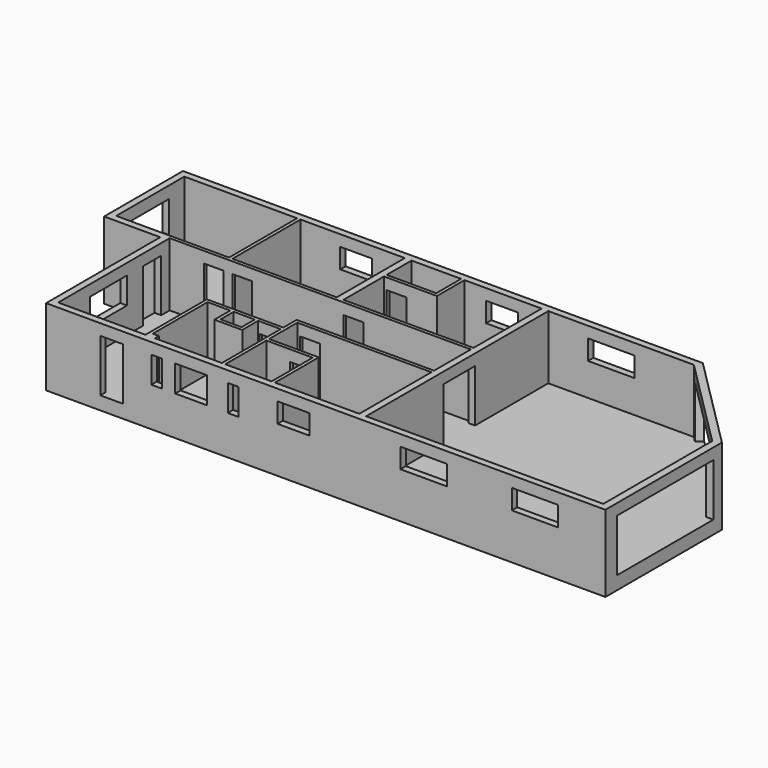
from build123d import *

# Parameters (mm, degrees)
F0_W          = 1750
F0_H          = 1938.4325688744
F0_W_2        = 796
F0_H_2        = 623
F0_W_3        = 4260
F0_H_3        = 3212
F0_W_4        = 3940
F0_W_5        = 1873
F0_H_4        = 1173
F1_DEPTH      = 2400
F1_DEPTH_BACK = 500
F2_W          = 750
F2_H          = 1980
F3_DEPTH      = 250
F4_W          = 750
F4_H          = 1980
F5_DEPTH      = 500
F6_W          = 750
F6_H          = 1980
F7_DEPTH      = 500
F8_W          = 1500
F8_H          = 1980
F9_DEPTH      = 500
F12_DEPTH     = 500
F13_W         = 750
F13_H         = 1980
F14_DEPTH     = 500
F15_W         = 1750
F15_H         = 1000
F15_W_2       = 850
F15_H_2       = 1980
F16_DEPTH     = 2374.001
F17_W         = 1750
F17_H         = 1200
F18_DEPTH     = 254.001
F19_W         = 850
F19_H         = 1980
F20_DEPTH     = 254.001
F21_W         = 400
F21_H         = 1000
F21_W_2       = 1200
F21_H_2       = 750
F21_W_3       = 1750
F22_DEPTH     = 254.001
F23_W         = 1200
F23_H         = 750
F23_W_2       = 1750
F24_DEPTH     = 254.001
F25_W         = 4294.8904704813
F25_H         = 1980
F26_DEPTH     = 2827.5745303553
F27_W         = 4540.7897551572
F27_H         = 1980
F28_DEPTH     = 283.5835903928
F29_W         = 750
F29_H         = 1980
F30_DEPTH     = 500


# Not quite as in the source:
# - a feature names something its author has since deleted; it is built from what else it names


with BuildPart() as f1:
    # F0 (on Top) → F1 (new body, two sides)
    with BuildSketch(Plane.XY) as f1_sk:
        Polygon((105.2102448428, 99.540888462), (-19524.7897551572, 99.540888462), (-19524.7897551572, -3620.459111538), (-17404.7897551572, -3620.459111538), (-17404.7897551572, -9010.459111538), (3715.2102448428, -9010.459111538), (3715.2102448428, -3510.459111538), align=None)
        Polygon((-13498.7586669922, -8566.459111538), (-13728.7586669922, -8566.459111538), (-13728.7586669922, -5983.459111538), (-12868.7586669922, -5983.459111538), (-12868.7586669922, -6733.459111538), (-11818.7586669922, -6733.459111538), (-11818.7586669922, -5983.459111538), (-10968.7586669922, -5983.459111538), (-10968.7586669922, -8756.459111538), (-13498.7586669922, -8756.459111538), align=None, mode=Mode.SUBTRACT)
        with Locations((-9966.7586669922, -7787.2428271008)):
            Rectangle(F0_W, F0_H, mode=Mode.SUBTRACT)
        Polygon((-10841.7586669922, -5356.459111538), (-5778.7897551572, -5356.459111538), (-5778.7897551572, -8756.459111538), (-8964.7586669922, -8756.459111538), (-8964.7586669922, -6691.0265426636), (-10841.7586669922, -6691.0265426636), align=None, mode=Mode.SUBTRACT)
        with Locations((-12343.7586669922, -6294.959111538)):
            Rectangle(F0_W_2, F0_H_2, mode=Mode.SUBTRACT)
        Polygon((-13855.7586669922, -8756.459111538), (-17150.7897551572, -8756.459111538), (-17150.7897551572, -3493.459111538), (-5778.7897551572, -3493.459111538), (-5778.7897551572, -5229.459111538), (-10968.7586669922, -5229.459111538), (-10968.7586669922, -5856.459111538), (-13855.7586669922, -5856.459111538), align=None, mode=Mode.SUBTRACT)
        Polygon((-5524.7897551572, -8756.459111538), (-5524.7897551572, -154.459111538), (-29.5825903928, -154.459111538), (3431.6276544499, -3615.6693563807), (3431.6276544499, -8756.459111538), align=None, mode=Mode.SUBTRACT)
        with Locations((-17140.7897551572, -1760.459111538)):
            Rectangle(F0_W_3, F0_H_3, mode=Mode.SUBTRACT)
        with Locations((-12913.7897551572, -1760.459111538)):
            Rectangle(F0_W_4, F0_H_3, mode=Mode.SUBTRACT)
        Polygon((-8689.7897551572, -154.459111538), (-5778.7897551572, -154.459111538), (-5778.7897551572, -3366.459111538), (-10689.7897551572, -3366.459111538), (-10689.7897551572, -1454.459111538), (-8689.7897551572, -1454.459111538), align=None, mode=Mode.SUBTRACT)
        with Locations((-9753.2897551572, -740.959111538)):
            Rectangle(F0_W_5, F0_H_4, mode=Mode.SUBTRACT)
    extrude(amount=F1_DEPTH)
    extrude(f1_sk.sketch, amount=-F1_DEPTH_BACK)

    # F2 (on face) → F3 (cut)
    with BuildSketch(Plane(origin=(0, -5856.459111538, 0), x_dir=(-1, 0, 0), z_dir=(0, 1, 0))):
        with Locations((11393.7586669922, 990)):
            Rectangle(F2_W, F2_H)
        with Locations((12343.7586669922, 490)):
            Rectangle(F2_W, F2_H)
    extrude(amount=-F3_DEPTH, mode=Mode.SUBTRACT)

    # F4 (on face) → F5 (cut)
    with BuildSketch(Plane.XZ.offset(3493.459111538)):
        with Locations((-15485.7897551572, 990)):
            Rectangle(F4_W, F4_H)
        with Locations((-14408.7897551572, 990)):
            Rectangle(F4_W, F4_H)
        with Locations((-10214.7897551572, 990)):
            Rectangle(F4_W, F4_H)
    extrude(amount=-F5_DEPTH, mode=Mode.SUBTRACT)

    # F6 (on face) → F7 (cut)
    with BuildSketch(Plane.XZ.offset(5356.459111538)):
        with Locations((-10366.7586669922, 990)):
            Rectangle(F6_W, F6_H)
    extrude(amount=-F7_DEPTH, mode=Mode.SUBTRACT)

    # F8 (on face) → F9 (cut)
    with BuildSketch(Plane(origin=(-5778.7897551572, 0, 0), x_dir=(0, -1, 0), z_dir=(-1, 0, 0))):
        with Locations((4361.459111538, 990)):
            Rectangle(F8_W, F8_H)
    extrude(amount=-F9_DEPTH, mode=Mode.SUBTRACT)

    # F11 (on face) → F12 (join)
    with BuildSketch(Plane(origin=(0, 0, -500), x_dir=(1, 0, 0), z_dir=(0, 0, -1))):
        Polygon((3715.2102448428, 3510.459111538), (3715.2102448428, 9010.459111538), (-17404.7897551572, 9010.459111538), (-17404.7897551572, 3620.459111538), (-19524.7897551572, 3620.459111538), (-19524.7897551572, -99.540888462), (105.2102448428, -99.540888462), align=None)
    extrude(amount=-F12_DEPTH)

    # F13 (on face) → F14 (cut)
    with BuildSketch(Plane.XZ.offset(6818.0265426636)):
        with Locations((-9566.7586669922, 990)):
            Rectangle(F13_W, F13_H)
    extrude(amount=-F14_DEPTH, mode=Mode.SUBTRACT)

    # F15 (on face) → F16 (cut, through all)
    with BuildSketch(Plane.YZ.offset(-17150.7897551572)):
        with Locations((-6381.459111538, 1480)):
            Rectangle(F15_W, F15_H)
        with Locations((-4318.459111538, 990)):
            Rectangle(F15_W_2, F15_H_2)
    extrude(amount=-F16_DEPTH, mode=Mode.SUBTRACT)

    # F17 (on face) → F18 (cut, through all)
    with BuildSketch(Plane.YZ.offset(-19270.7897551572)):
        with Locations((-1741.459111538, 1350)):
            Rectangle(F17_W, F17_H)
    extrude(amount=-F18_DEPTH, mode=Mode.SUBTRACT)

    # F19 (on face) → F20 (cut, through all)
    with BuildSketch(Plane(origin=(0, -8756.459111538, 0), x_dir=(-1, 0, 0), z_dir=(0, 1, 0))):
        with Locations((14930.7586669922, 990)):
            Rectangle(F19_W, F19_H)
    extrude(amount=-F20_DEPTH, mode=Mode.SUBTRACT)

    # F21 (on face) → F22 (cut, through all)
    with BuildSketch(Plane(origin=(0, -8756.459111538, 0), x_dir=(-1, 0, 0), z_dir=(0, 1, 0))):
        with Locations((13228.7586669922, 1480)):
            Rectangle(F21_W, F21_H)
        with Locations((11928.7586669922, 1480)):
            Rectangle(F21_W_2, F21_H)
        with Locations((10341.7586669922, 1480)):
            Rectangle(F21_W, F21_H)
        with Locations((8064.7586669922, 1605)):
            Rectangle(F21_W_2, F21_H_2)
        with Locations((3149.7897551572, 1605)):
            Rectangle(F21_W_3, F21_H_2)
        with Locations((-1056.6276544499, 1605)):
            Rectangle(F21_W_3, F21_H_2)
    extrude(amount=-F22_DEPTH, mode=Mode.SUBTRACT)

    # F23 (on face) → F24 (cut, through all)
    with BuildSketch(Plane.XZ.offset(154.459111538)):
        with Locations((-12783.7897551572, 1605)):
            Rectangle(F23_W, F23_H)
        with Locations((-7278.7897551572, 1605)):
            Rectangle(F23_W, F23_H)
        with Locations((-3149.7897551572, 1605)):
            Rectangle(F23_W_2, F23_H)
    extrude(amount=-F24_DEPTH, mode=Mode.SUBTRACT)

    # F25 (on face) → F26 (cut, through all)
    with BuildSketch(Plane(origin=(-92.0208509654, -92.0208509654, 0), x_dir=(0.7071067812, -0.7071067812, 0), z_dir=(-0.7071067812, -0.7071067812, 0))):
        with Locations((2535.7462701534, 990)):
            Rectangle(F25_W, F25_H)
    extrude(amount=-F26_DEPTH, mode=Mode.SUBTRACT)

    # F27 (on face) → F28 (cut, through all)
    with BuildSketch(Plane(origin=(3431.6276544499, 0, 0), x_dir=(0, -1, 0), z_dir=(-1, 0, 0))):
        with Locations((6186.0642339594, 990)):
            Rectangle(F27_W, F27_H)
    extrude(amount=-F28_DEPTH, mode=Mode.SUBTRACT)

    # F29 (on face) → F30 (cut)
    with BuildSketch(Plane.XZ.offset(1454.459111538)):
        with Locations((-10214.7897551572, 990)):
            Rectangle(F29_W, F29_H)
    extrude(amount=-F30_DEPTH, mode=Mode.SUBTRACT)


solid = f1.part
